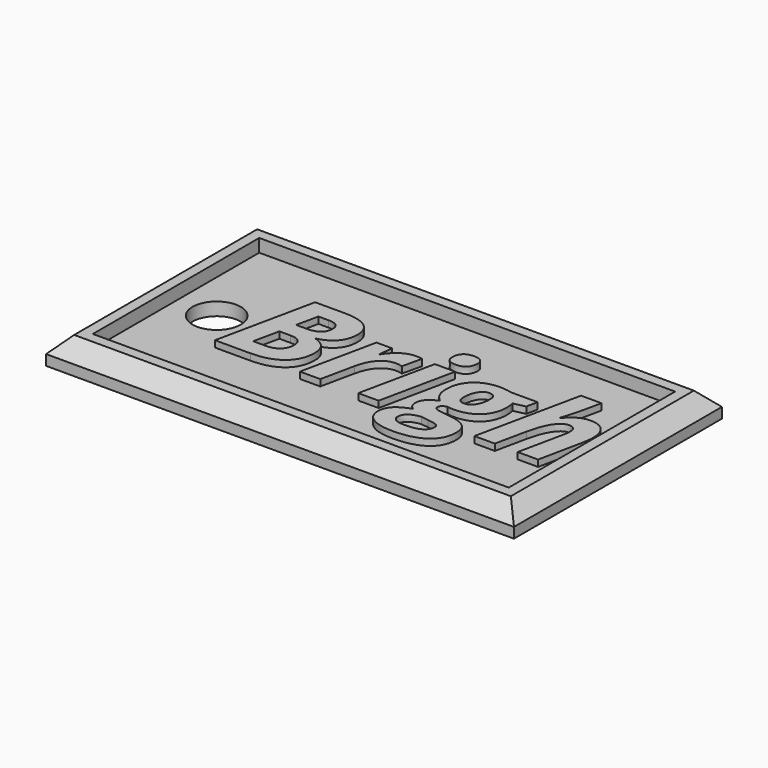
from build123d import *

# Parameters (mm, degrees)
F0_W         = 50.8
F0_H         = 25.4
F0_R         = 2.9459153188
F1_DEPTH     = 1.5875
F0_W_2       = 57.15
F0_H_2       = 31.75
F2_DEPTH     = 3.175
F3_SIZE      = 1.905
F4_TEXT_SIZE = 16.9333333333
F6_DEPTH     = 0.79375


# Not quite as in the source:
# - Text() gives the source's letters only with a copy of the font that has no kerning and outlines rounded to 1/6400 em; it was checked with that copy


with BuildPart() as f1:
    # F0 (on Top) → F1 (new body)
    with BuildSketch(Plane.XY):
        with Locations((25.4, 12.7)):
            Rectangle(F0_W, F0_H)
        with Locations((4.9641244113, 12.7)):
            Circle(F0_R, mode=Mode.SUBTRACT)
    extrude(amount=F1_DEPTH)

    # F0 (on Top) → F2 (join)
    with BuildSketch(Plane.XY):
        with Locations((25.4, 12.7)):
            Rectangle(F0_W_2, F0_H_2)
        with Locations((25.4, 12.7)):
            Rectangle(F0_W, F0_H, mode=Mode.SUBTRACT)
    extrude(amount=F2_DEPTH)

    # F3
    f3_edges = [f1.edges().sort_by_distance(p)[0] for p in [
        (25.4, -3.175, 3.175),
        (-3.175, 12.7, 3.175),
        (25.4, 28.575, 3.175),
        (53.975, 12.7, 3.175),
    ]]
    chamfer(f3_edges, length=F3_SIZE)

    # F4 (on face) → F6 (join)
    with BuildSketch(Plane.XY.offset(1.5875)):
        with Locations((8.5142916667, 7.4565670932)):
            Text('Brigh', F4_TEXT_SIZE, font='Open Sans', font_style=FontStyle.BOLDITALIC, text_align=(TextAlign.LEFT, TextAlign.BOTTOM))
    extrude(amount=F6_DEPTH)


solid = f1.part
